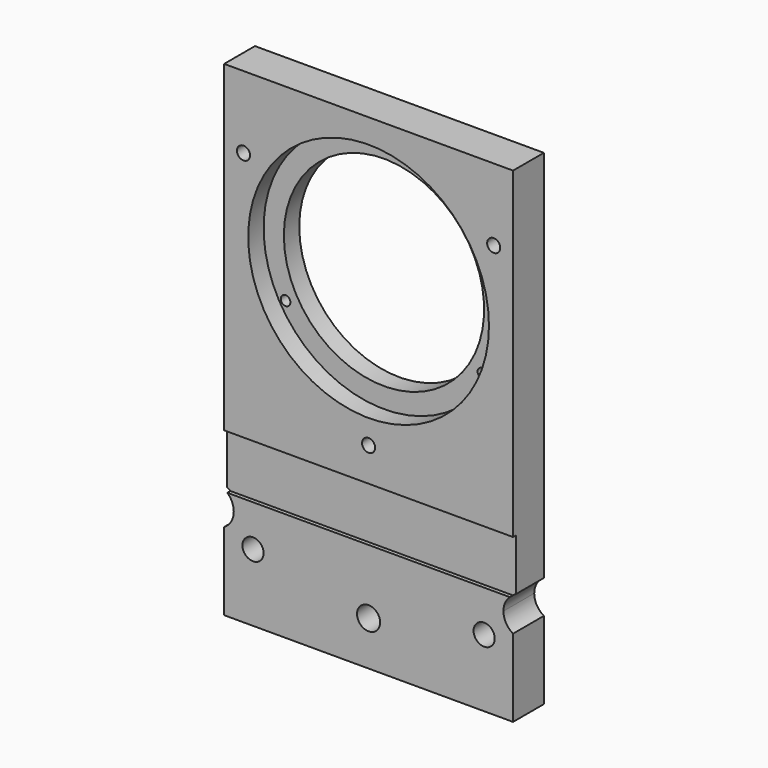
from build123d import *

# Parameters (mm, degrees)
F0_W             = 150
F0_H             = 90
F1_DEPTH         = 20
F2_R             = 5.5
F3_DEPTH         = 20.001
F4_W             = 2
F4_H             = 28
F5_DEPTH         = 150.001
F6_W             = 150
F6_H             = 124
F6_R             = 30
F7_DEPTH         = 20
F9_DEPTH         = 20.001
F11_W            = 150
F11_H            = 20
F12_DEPTH        = 20
F13_R            = 6
F14_DEPTH        = 20.001
F15_W            = 150
F15_H            = 18
F16_DEPTH        = 20
F17_R            = 52
F17_R_2          = 30
F18_DEPTH        = 20
F20_R            = 62.5
F20_R_2          = 52
F21_DEPTH        = 10
F22_R            = 3.4
F23_DEPTH        = 20.001
F23_COPIES_COUNT = 3
F24_R            = 2.5
F25_DEPTH        = 20.001
F25_COPIES_COUNT = 3


# Not quite as in the source:
# - a pattern or mirror of a feature is missing from the dataset's text; its kind, count and spacing are read off the source's solid


with BuildPart() as f1:
    # F0 (on Front) → F1 (new body)
    with BuildSketch(Plane.XZ):
        with Locations((0, -15)):
            Rectangle(F0_W, F0_H)
    extrude(amount=F1_DEPTH)

    # F2 (on face) → F3 (cut, through all)
    with BuildSketch(Plane.XZ.offset(20)):
        with Locations((-60, -45)):
            Circle(F2_R)
        with Locations((60, -45)):
            Circle(F2_R)
    extrude(amount=-F3_DEPTH, mode=Mode.SUBTRACT)

    # F4 (on face) → F5 (cut, through all)
    with BuildSketch(Plane(origin=(-75, 0, 0), x_dir=(0, -1, 0), z_dir=(-1, 0, 0))):
        with Locations((19, -9.5)):
            Rectangle(F4_W, F4_H)
    extrude(amount=-F5_DEPTH, mode=Mode.SUBTRACT)

    # F6 (on face) → F7 (join)
    with BuildSketch(Plane(origin=(0, 0, 0), x_dir=(-1, 0, 0), z_dir=(0, 1, 0))):
        with Locations((0, 92)):
            Rectangle(F6_W, F6_H)
        with Locations((0, 97)):
            Circle(F6_R, mode=Mode.SUBTRACT)
    extrude(amount=-F7_DEPTH)

    # F8 (on face) → F9 (cut, through all)
    with BuildSketch(Plane(origin=(0, 0, 0), x_dir=(-1, 0, 0), z_dir=(0, 1, 0))):
        with BuildLine():
            ThreePointArc((-75, -39.6602540378), (-71.3397459622, -36), (-70, -31))
            ThreePointArc((-70, -31), (-71.3397459622, -26), (-75, -22.3397459622))
            Line((-75, -22.3397459622), (-75, -39.6602540378))
        make_face()
        with BuildLine():
            Line((-75, -39.6602540378), (-75, -22.3397459622))
            ThreePointArc((-75, -22.3397459622), (-90, -31), (-75, -39.6602540378))
        make_face()
        with BuildLine():
            Line((75, -39.6602540378), (75, -22.3397459622))
            ThreePointArc((75, -22.3397459622), (70, -31), (75, -39.6602540378))
        make_face()
        with BuildLine():
            ThreePointArc((90, -31), (85, -22.3397459622), (75, -22.3397459622))
            Line((75, -22.3397459622), (75, -39.6602540378))
            ThreePointArc((75, -39.6602540378), (85, -39.6602540378), (90, -31))
        make_face()
    extrude(amount=-F9_DEPTH, mode=Mode.SUBTRACT)

    # F11 (on face) → F12 (join)
    with BuildSketch(Plane(origin=(0, 0, 0), x_dir=(-1, 0, 0), z_dir=(0, 1, 0))):
        with Locations((0, -70)):
            Rectangle(F11_W, F11_H)
    extrude(amount=-F12_DEPTH)

    # F13 (on face) → F14 (cut, through all)
    with BuildSketch(Plane(origin=(0, 0, 0), x_dir=(-1, 0, 0), z_dir=(0, 1, 0))):
        with Locations((0, -57)):
            Circle(F13_R)
    extrude(amount=-F14_DEPTH, mode=Mode.SUBTRACT)

    # F15 (on face) → F16 (join)
    with BuildSketch(Plane.XZ.offset(20)):
        with Locations((0, 163)):
            Rectangle(F15_W, F15_H)
    extrude(amount=-F16_DEPTH)

    # F17 (on face) → F18 (cut)
    with BuildSketch(Plane(origin=(0, 0, 0), x_dir=(-1, 0, 0), z_dir=(0, 1, 0))):
        with Locations((0, 97)):
            Circle(F17_R)
        with Locations((0, 97)):
            Circle(F17_R_2, mode=Mode.SUBTRACT)
    extrude(amount=-F18_DEPTH, mode=Mode.SUBTRACT)

    # F20 (on face) → F21 (cut)
    with BuildSketch(Plane.XZ.offset(20)):
        with Locations((0, 97)):
            Circle(F20_R)
        with Locations((0, 97)):
            Circle(F20_R_2, mode=Mode.SUBTRACT)
    extrude(amount=-F21_DEPTH, mode=Mode.SUBTRACT)

    # F22 (on face) → F23 (cut, through all)
    with BuildSketch(Plane.XZ.offset(20)):
        with Locations((0, 22)):
            Circle(F22_R)
    f23 = extrude(amount=-F23_DEPTH, mode=Mode.SUBTRACT)

    # F23_copies: F23 ×3 about axis
    f23_copies_axis = Axis((0, 0, 97), (0, 1, 0))
    for i in range(1, F23_COPIES_COUNT):
        add(f23.rotate(f23_copies_axis, i * 360 / F23_COPIES_COUNT), mode=Mode.SUBTRACT)

    # F24 (on face) → F25 (cut, through all)
    with BuildSketch(Plane(origin=(0, 0, 0), x_dir=(-1, 0, 0), z_dir=(0, 1, 0))):
        with Locations((0, 156)):
            Circle(F24_R)
    f25 = extrude(amount=-F25_DEPTH, mode=Mode.SUBTRACT)

    # F25_copies: F25 ×3 about axis
    f25_copies_axis = Axis((0, 0, 97), (0, 1, 0))
    for i in range(1, F25_COPIES_COUNT):
        add(f25.rotate(f25_copies_axis, i * 360 / F25_COPIES_COUNT), mode=Mode.SUBTRACT)


solid = f1.part
